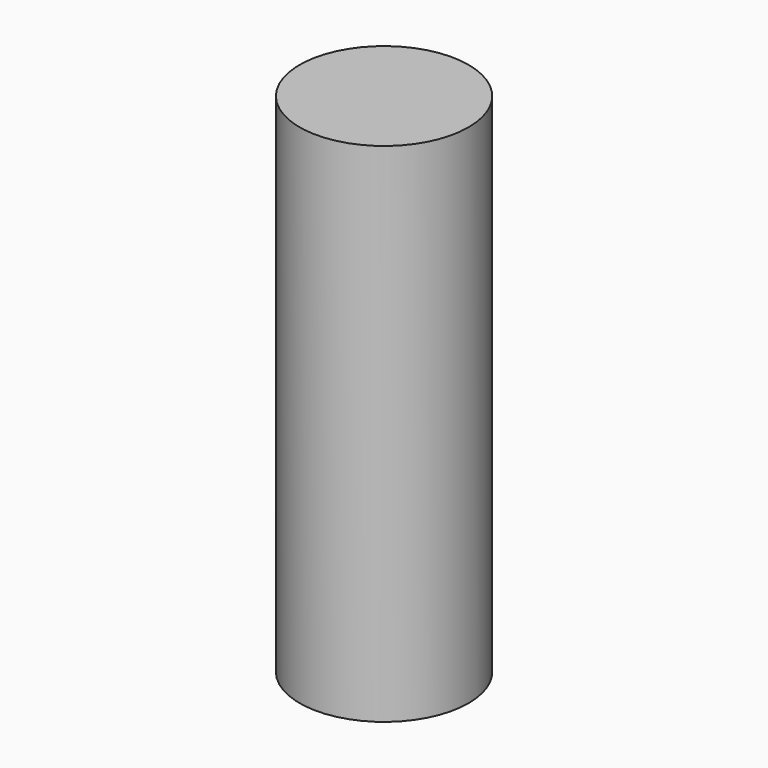
from build123d import *

# Parameters (mm, degrees)
F0_R     = 5
F1_DEPTH = 30
F2_R     = 4
F3_DEPTH = 28.5409297794


# Not quite as in the source:
# - a feature names something its author has since deleted; it is built from what else it names


with BuildPart() as f1:
    # F0 (on Top) → F1 (new body)
    with BuildSketch(Plane.XY):
        Circle(F0_R)
    extrude(amount=F1_DEPTH)

    # F2 (on face) → F3 (cut)
    with BuildSketch(Plane.XY):
        Circle(F2_R)
    extrude(amount=F3_DEPTH, mode=Mode.SUBTRACT)


solid = f1.part
